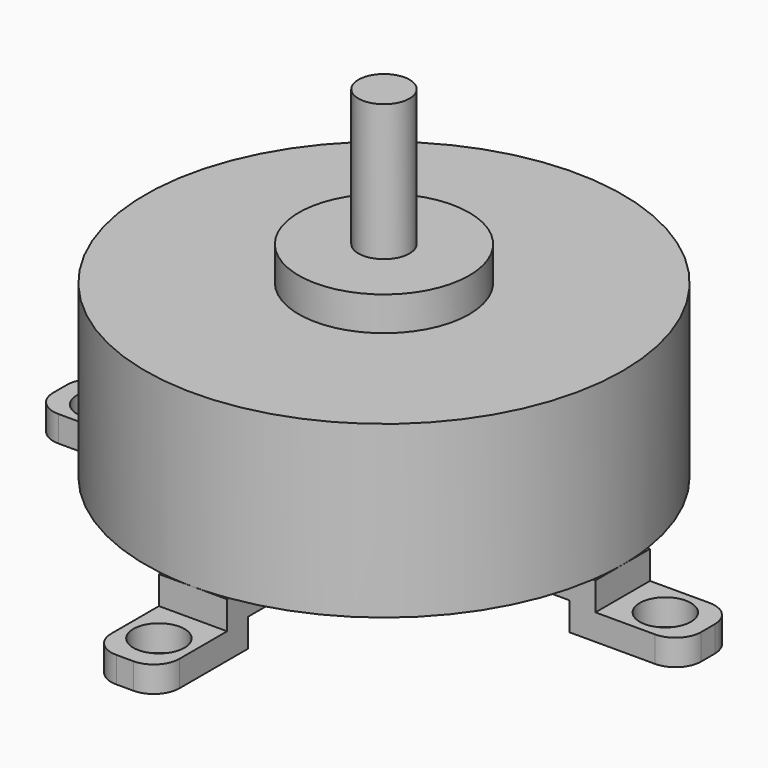
from build123d import *

# Parameters (mm, degrees)
F0_R     = 14
F1_DEPTH = 10
F2_R     = 5
F2_R_2   = 1.5
F3_DEPTH = 2
F4_DEPTH = 10
F5_W     = 5
F5_H     = 1.524
F6_DEPTH = 2
F7_R     = 1.5
F8_DEPTH = 25.4
F9_R     = 1.5


# Not quite as in the source:
# - a pattern or mirror of a feature is missing from the dataset's text; its kind, count and spacing are read off the source's solid


with BuildPart() as f1:
    # F0 (on Top) → F1 (new body)
    with BuildSketch(Plane.XY):
        Circle(F0_R)
    extrude(amount=F1_DEPTH)

    # F2 (on face) → F3 (join)
    with BuildSketch(Plane.XY.offset(10)):
        Circle(F2_R)
        Circle(F2_R_2, mode=Mode.SUBTRACT)
    extrude(amount=F3_DEPTH)

    # F4 (add): a face of the model
    f4_faces = [f1.faces().sort_by_distance(p)[0] for p in [
        (0, 0, 10),
    ]]
    extrude(f4_faces, amount=F4_DEPTH)

    # F5 (on Front) → F6 (join, symmetric)
    with BuildSketch(Plane.XZ):
        Polygon((14, 0), (-14, 0), (-14, -1.524), (-12.476, -1.524), (12.476, -1.524), (14, -1.524), align=None)
        Polygon((-12.476, -1.524), (-14, -1.524), (-14, -1.651), (-14, -3.175), (-12.476, -3.175), align=None)
        with Locations((-16.5, -2.413)):
            Rectangle(F5_W, F5_H)
        Polygon((14, -1.651), (14, -1.524), (12.476, -1.524), (12.476, -3.175), (14, -3.175), align=None)
        with Locations((16.5, -2.413)):
            Rectangle(F5_W, F5_H)
    f6 = extrude(amount=F6_DEPTH, both=True)

    # F6_copies: F6 across plane
    add(f6.mirror(Plane(origin=(0, 0, 0), x_dir=(-0.7071067812, -0.7071067812, 0), z_dir=(-0.7071067812, 0.7071067812, 0))))

    # F7 (on face) → F8 (cut)
    with BuildSketch(Plane.XY.offset(-1.651)):
        with Locations((-16.5, 0)):
            Circle(F7_R)
        with BuildLine():
            ThreePointArc((18, 0), (16.5, 1.5), (15, 0))
            ThreePointArc((15, 0), (16.5, -1.5), (18, 0))
        make_face()
    f8 = extrude(amount=-F8_DEPTH, mode=Mode.SUBTRACT)

    # F8_copies: F8 across plane
    add(f8.mirror(Plane(origin=(0, 0, 0), x_dir=(0.7071067812, 0.7071067812, 0), z_dir=(0.7071067812, -0.7071067812, 0))), mode=Mode.SUBTRACT)

    # F9
    f9_edges = [f1.edges().sort_by_distance(p)[0] for p in [
        (-19, -2, -2.413),
        (-19, 2, -2.413),
        (19, -2, -2.413),
        (19, 2, -2.413),
        (2, 19, -2.413),
        (-2, 19, -2.413),
        (-2, -19, -2.413),
        (2, -19, -2.413),
    ]]
    fillet(f9_edges, radius=F9_R)


solid = f1.part
